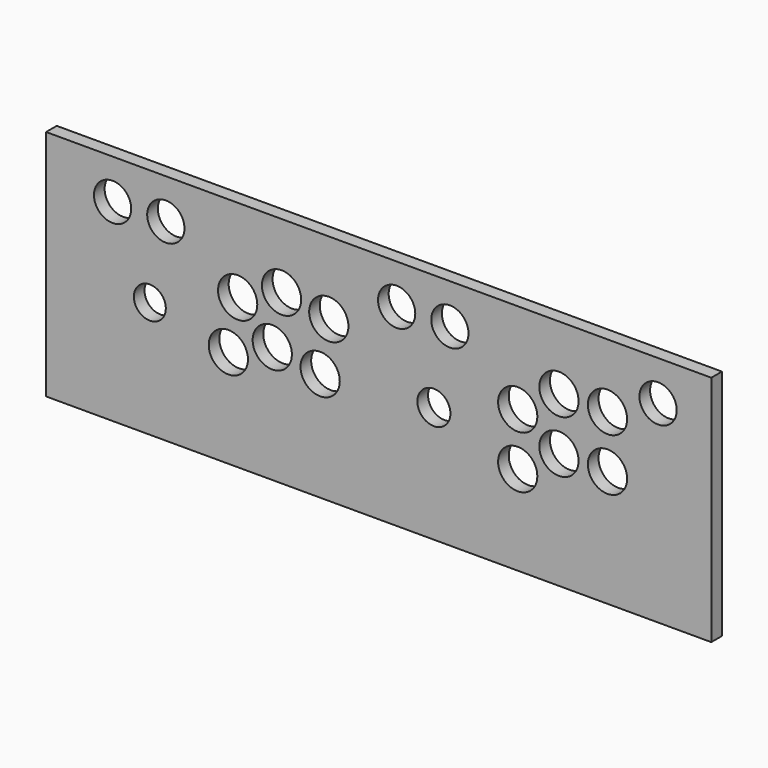
from build123d import *

# Parameters (mm, degrees)
F0_W     = 500
F0_H     = 175
F1_DEPTH = 10
F5_R     = 14.75
F5_R_2   = 12.4064380464
F7_DEPTH = 25
F3_R     = 14.75
F3_R_2   = 12
F8_DEPTH = 25
F6_R     = 14
F9_DEPTH = 25


# Not quite as in the source:
# - a feature names something its author has since deleted; it is built from what else it names


with BuildPart() as f1:
    # F0 (on Front) → F1 (new body)
    with BuildSketch(Plane.XZ):
        with Locations((250, 87.5)):
            Rectangle(F0_W, F0_H)
    extrude(amount=F1_DEPTH)

    # F5 (on face) → F7 (cut)
    with BuildSketch(Plane.XZ.offset(10)):
        with Locations((354.5, 106.75)):
            Circle(F5_R)
        with Locations((385.5, 127)):
            Circle(F5_R)
        with Locations((422, 127)):
            Circle(F5_R)
        with Locations((422, 87.5)):
            Circle(F5_R)
        with Locations((385.5, 87.5)):
            Circle(F5_R)
        with Locations((354.5, 67.25)):
            Circle(F5_R)
        with Locations((291.5, 87.5)):
            Circle(F5_R_2)
    extrude(amount=-F7_DEPTH, mode=Mode.SUBTRACT)

    # F3 (on face) → F8 (cut)
    with BuildSketch(Plane.XZ.offset(10)):
        with Locations((177, 126.3350188136)):
            Circle(F3_R)
        with Locations((212.5, 120.3350188136)):
            Circle(F3_R)
        with Locations((206, 81.8350188136)):
            Circle(F3_R)
        with Locations((170, 87.8350188136)):
            Circle(F3_R)
        with Locations((137, 73.8350188136)):
            Circle(F3_R)
        with Locations((144, 112.3350188136)):
            Circle(F3_R)
        with Locations((78, 87.5)):
            Circle(F3_R_2)
    extrude(amount=-F8_DEPTH, mode=Mode.SUBTRACT)

    # F6 (on face) → F9 (cut)
    with BuildSketch(Plane.XZ.offset(10)):
        with Locations((263.5, 145)):
            Circle(F6_R)
        with Locations((50, 145)):
            Circle(F6_R)
        with Locations((90, 145)):
            Circle(F6_R)
        with Locations((303.5, 145)):
            Circle(F6_R)
        with Locations((460, 145)):
            Circle(F6_R)
    extrude(amount=-F9_DEPTH, mode=Mode.SUBTRACT)


solid = f1.part
